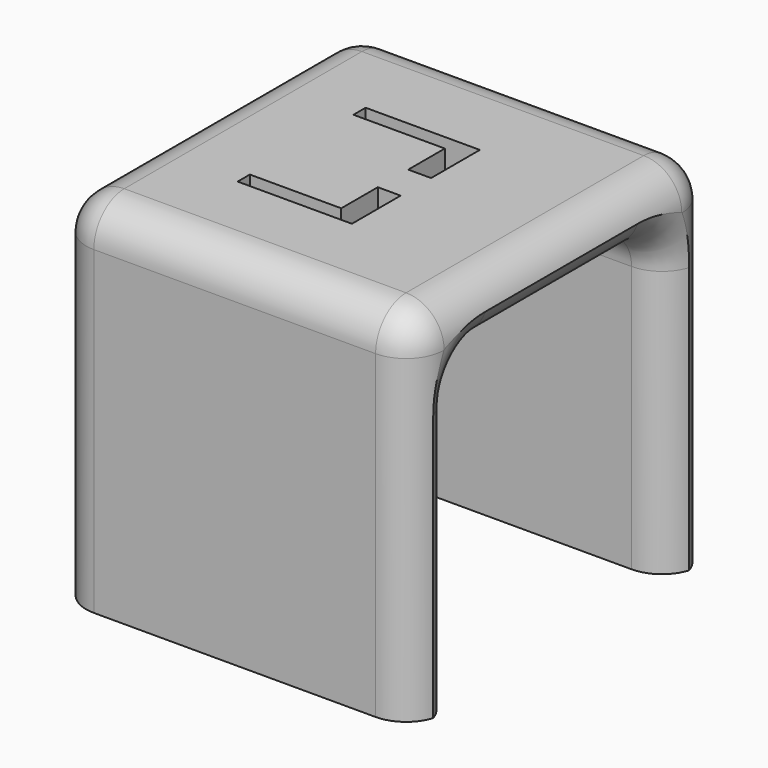
from build123d import *

# Parameters (mm, degrees)
F0_W         = 47
F0_H         = 47
F1_DEPTH     = 49
F3_DEPTH     = 40
F4_T1_DEPTH  = 37
F4_T3_DEPTH  = 54.5
F4_T5_DEPTH  = 39
F4_T7_DEPTH  = 25
F4_T9_DEPTH  = 47.5
F4_S13_W     = 5
F4_S13_H     = 5
F4_T14_DEPTH = 5
F4_S19_W     = 5
F4_S19_H     = 5
F4_T20_DEPTH = 5
F4_S25_W     = 5
F4_S25_H     = 5
F4_T26_DEPTH = 5
F4_S31_W     = 5
F4_S31_H     = 5
F4_T32_DEPTH = 5
F4_T36_ANGLE = 90
F4_T38_ANGLE = 90
F6_R         = 2.75
F7_DEPTH     = 21
F8_W         = 15
F8_H         = 21
F9_DEPTH     = 4
F10_W        = 3
F10_H        = 6
F10_W_2      = 12
F10_H_2      = 2
F11_DEPTH    = 3.0010001


# Not quite as in the source:
# - a fillet or chamfer that OpenCascade refuses, or shapes differently, is made with other operations: its cross-section is extruded or revolved along the edge and cut away or added


with BuildPart() as f1:
    # F0 (on Front) → F1 (new body)
    with BuildSketch(Plane.XZ):
        with Locations((-31.9517639409, 6.0313746929)):
            Rectangle(F0_W, F0_H)
    extrude(amount=F1_DEPTH)

    # F2 (on face) → F3 (cut)
    with BuildSketch(Plane.YZ.offset(-8.4517639409)):
        with BuildLine():
            Line((-12, 22.5313746929), (-37, 22.5313746929))
            ThreePointArc((-37, 22.5313746929), (-40.5355339059, 21.0669085988), (-42, 17.5313746929))
            Line((-42, 17.5313746929), (-42, -17.4686253071))
            Line((-42, -17.4686253071), (-7, -17.4686253071))
            Line((-7, -17.4686253071), (-7, 17.5313746929))
            ThreePointArc((-7, 17.5313746929), (-8.4644660941, 21.0669085988), (-12, 22.5313746929))
        make_face()
    extrude(amount=-F3_DEPTH, mode=Mode.SUBTRACT)

    # F4: fillet of radius 5 on 9 edges, made by hand

    # F4_s2 → F4_t1 (cut)
    with BuildSketch(Plane.YZ.offset(-50.4517639409)):
        with BuildLine():
            ThreePointArc((-44, 29.5313746929), (-47.5355339059, 28.0669085988), (-49, 24.5313746929))
            Line((-49, 24.5313746929), (-49, 29.5313746929))
            Line((-49, 29.5313746929), (-44, 29.5313746929))
        make_face()
        with BuildLine():
            ThreePointArc((0, 24.5313746929), (-1.4644660941, 28.0669085988), (-5, 29.5313746929))
            Line((-5, 29.5313746929), (0, 29.5313746929))
            Line((0, 29.5313746929), (0, 24.5313746929))
        make_face()
    extrude(amount=F4_T1_DEPTH, mode=Mode.SUBTRACT)

    # F4_s4 → F4_t3 (cut)
    with BuildSketch(Plane.XY.offset(-29.9686253071)):
        with BuildLine():
            ThreePointArc((-8.4517639409, -44), (-9.9162300349, -47.5355339059), (-13.4517639409, -49))
            Line((-13.4517639409, -49), (-8.4517639409, -49))
            Line((-8.4517639409, -49), (-8.4517639409, -44))
        make_face()
        with BuildLine():
            ThreePointArc((-8.4517639409, -5), (-9.9162300349, -1.4644660941), (-13.4517639409, 0))
            Line((-13.4517639409, 0), (-8.4517639409, 0))
            Line((-8.4517639409, 0), (-8.4517639409, -5))
        make_face()
        with BuildLine():
            ThreePointArc((-50.4517639409, 0), (-53.9872978468, -1.4644660941), (-55.4517639409, -5))
            Line((-55.4517639409, -5), (-55.4517639409, 0))
            Line((-55.4517639409, 0), (-50.4517639409, 0))
        make_face()
        with BuildLine():
            ThreePointArc((-50.4517639409, -49), (-53.9872978468, -47.5355339059), (-55.4517639409, -44))
            Line((-55.4517639409, -44), (-55.4517639409, -49))
            Line((-55.4517639409, -49), (-50.4517639409, -49))
        make_face()
    extrude(amount=F4_T3_DEPTH, mode=Mode.SUBTRACT)

    # F4_s6 → F4_t5 (cut)
    with BuildSketch(Plane.XZ.offset(5)):
        with BuildLine():
            ThreePointArc((-8.4517639409, 24.5313746929), (-9.9162300349, 28.0669085988), (-13.4517639409, 29.5313746929))
            Line((-13.4517639409, 29.5313746929), (-8.4517639409, 29.5313746929))
            Line((-8.4517639409, 29.5313746929), (-8.4517639409, 24.5313746929))
        make_face()
        with BuildLine():
            ThreePointArc((-50.4517639409, 29.5313746929), (-53.9872978468, 28.0669085988), (-55.4517639409, 24.5313746929))
            Line((-55.4517639409, 24.5313746929), (-55.4517639409, 29.5313746929))
            Line((-55.4517639409, 29.5313746929), (-50.4517639409, 29.5313746929))
        make_face()
    extrude(amount=F4_T5_DEPTH, mode=Mode.SUBTRACT)

    # F4_s8 → F4_t7 (cut)
    with BuildSketch(Plane.XZ.offset(12)):
        with BuildLine():
            ThreePointArc((-8.4517639409, 27.5313746929), (-9.9162300349, 23.995840787), (-13.4517639409, 22.5313746929))
            Line((-13.4517639409, 22.5313746929), (-8.4517639409, 22.5313746929))
            Line((-8.4517639409, 22.5313746929), (-8.4517639409, 27.5313746929))
        make_face()
    extrude(amount=F4_T7_DEPTH, mode=Mode.SUBTRACT)

    # F4_s10 → F4_t9 (cut)
    with BuildSketch(Plane.XY.offset(-29.9686253071)):
        with BuildLine():
            ThreePointArc((-8.4517639409, -47), (-9.9162300349, -43.4644660941), (-13.4517639409, -42))
            Line((-13.4517639409, -42), (-8.4517639409, -42))
            Line((-8.4517639409, -42), (-8.4517639409, -47))
        make_face()
        with BuildLine():
            ThreePointArc((-8.4517639409, -2), (-9.9162300349, -5.5355339059), (-13.4517639409, -7))
            Line((-13.4517639409, -7), (-8.4517639409, -7))
            Line((-8.4517639409, -7), (-8.4517639409, -2))
        make_face()
    extrude(amount=F4_T9_DEPTH, mode=Mode.SUBTRACT)


with BuildPart() as f4_tool12:
    # F4_s13 → F4_t14 (new body)
    with BuildSketch(Plane.YZ.offset(-13.4517639409)):
        with Locations((-46.5, 27.0313746929)):
            Rectangle(F4_S13_W, F4_S13_H)
    extrude(amount=F4_T14_DEPTH)

    # F4_s15 → F4_t16 (revolve, cut)
    with BuildSketch(Plane(origin=(-13.4517639409, -44, 24.5313746929), x_dir=(0, 0.7071067812, -0.7071067812), z_dir=(0, -0.7071067812, -0.7071067812))):
        with BuildLine():
            ThreePointArc((0, -5), (5, 0), (0, 5))
            Line((0, 5), (0, -5))
        make_face()
    revolve(axis=Axis((-13.4517639409, -44, 24.5313746929), (1, 0, 0)), mode=Mode.SUBTRACT)


with BuildPart() as f1_1:
    add(f1.part)

    # F4_t11: cut F4_tool12
    add(f4_tool12.part, mode=Mode.SUBTRACT)


with BuildPart() as f4_tool18:
    # F4_s19 → F4_t20 (new body)
    with BuildSketch(Plane.YZ.offset(-50.4517639409)):
        with Locations((-46.5, 27.0313746929)):
            Rectangle(F4_S19_W, F4_S19_H)
    extrude(amount=-F4_T20_DEPTH)

    # F4_s21 → F4_t22 (revolve, cut)
    with BuildSketch(Plane(origin=(-50.4517639409, -44, 24.5313746929), x_dir=(0, 0.7071067812, -0.7071067812), z_dir=(0, 0.7071067812, 0.7071067812))):
        with BuildLine():
            ThreePointArc((0, -5), (5, 0), (0, 5))
            Line((0, 5), (0, -5))
        make_face()
    revolve(axis=Axis((-50.4517639409, -44, 24.5313746929), (-1, 0, 0)), mode=Mode.SUBTRACT)


with BuildPart() as f1_2:
    add(f1_1.part)

    # F4_t17: cut F4_tool18
    add(f4_tool18.part, mode=Mode.SUBTRACT)


with BuildPart() as f4_tool24:
    # F4_s25 → F4_t26 (new body)
    with BuildSketch(Plane.YZ.offset(-13.4517639409)):
        with Locations((-2.5, 27.0313746929)):
            Rectangle(F4_S25_W, F4_S25_H)
    extrude(amount=F4_T26_DEPTH)

    # F4_s27 → F4_t28 (revolve, cut)
    with BuildSketch(Plane(origin=(-13.4517639409, -5, 24.5313746929), x_dir=(0, -0.7071067812, -0.7071067812), z_dir=(0, -0.7071067812, 0.7071067812))):
        with BuildLine():
            ThreePointArc((0, -5), (5, 0), (0, 5))
            Line((0, 5), (0, -5))
        make_face()
    revolve(axis=Axis((-13.4517639409, -5, 24.5313746929), (1, 0, 0)), mode=Mode.SUBTRACT)


with BuildPart() as f1_3:
    add(f1_2.part)

    # F4_t23: cut F4_tool24
    add(f4_tool24.part, mode=Mode.SUBTRACT)


with BuildPart() as f4_tool30:
    # F4_s31 → F4_t32 (new body)
    with BuildSketch(Plane.XZ.offset(5)):
        with Locations((-52.9517639409, 27.0313746929)):
            Rectangle(F4_S31_W, F4_S31_H)
    extrude(amount=-F4_T32_DEPTH)

    # F4_s33 → F4_t34 (revolve, cut)
    with BuildSketch(Plane(origin=(-50.4517639409, -5, 24.5313746929), x_dir=(0.7071067812, 0, -0.7071067812), z_dir=(0.7071067812, 0, 0.7071067812))):
        with BuildLine():
            ThreePointArc((0, -5), (5, 0), (0, 5))
            Line((0, 5), (0, -5))
        make_face()
    revolve(axis=Axis((-50.4517639409, -5, 24.5313746929), (0, 1, 0)), mode=Mode.SUBTRACT)


with BuildPart() as f1_4:
    add(f1_3.part)

    # F4_t29: cut F4_tool30
    add(f4_tool30.part, mode=Mode.SUBTRACT)

    # F4_s35 → F4_t36 (revolve, cut)
    with BuildSketch(Plane.XY.offset(17.5313746929)):
        with BuildLine():
            ThreePointArc((-8.4517639409, -2), (-9.9162300349, -5.5355339059), (-13.4517639409, -7))
            Line((-13.4517639409, -7), (-8.4517639409, -7))
            Line((-8.4517639409, -7), (-8.4517639409, -2))
        make_face()
    revolve(axis=Axis((-8.4517639409, -12, 17.5313746929), (1, 0, 0)), revolution_arc=F4_T36_ANGLE, mode=Mode.SUBTRACT)

    # F4_s37 → F4_t38 (revolve, cut)
    with BuildSketch(Plane.XZ.offset(37)):
        with BuildLine():
            ThreePointArc((-8.4517639409, 27.5313746929), (-9.9162300349, 23.995840787), (-13.4517639409, 22.5313746929))
            Line((-13.4517639409, 22.5313746929), (-8.4517639409, 22.5313746929))
            Line((-8.4517639409, 22.5313746929), (-8.4517639409, 27.5313746929))
        make_face()
    revolve(axis=Axis((-8.4517639409, -37, 17.5313746929), (1, 0, 0)), revolution_arc=F4_T38_ANGLE, mode=Mode.SUBTRACT)

    # F6 (on offset) → F7 (cut)
    with BuildSketch(Plane.XZ.offset(14.5)):
        with Locations((-45.4517639409, 24.5701503009)):
            Circle(F6_R)
    extrude(amount=F7_DEPTH, mode=Mode.SUBTRACT)

    # F8 (on face) → F9 (cut)
    with BuildSketch(Plane(origin=(0, 0, 22.5313746929), x_dir=(1, 0, 0), z_dir=(0, 0, -1))):
        with Locations((-34.8641358682, 25)):
            Rectangle(F8_W, F8_H)
    extrude(amount=-F9_DEPTH, mode=Mode.SUBTRACT)

    # F10 (on face) → F11 (cut, through all)
    with BuildSketch(Plane(origin=(0, 0, 26.5313746929), x_dir=(1, 0, 0), z_dir=(0, 0, -1))):
        with Locations((-28.8641358682, 30.5)):
            Rectangle(F10_W, F10_H)
        Polygon((-30.3641358682, 22.5), (-30.3641358682, 16.5), (-30.3641358682, 14.5), (-27.3641358682, 14.5), (-27.3641358682, 22.5), align=None)
        with Locations((-36.3641358682, 34.5)):
            Rectangle(F10_W_2, F10_H_2)
        with Locations((-28.8641358682, 34.5)):
            Rectangle(F10_W, F10_H_2)
        with Locations((-36.3641358682, 15.5)):
            Rectangle(F10_W_2, F10_H_2)
    extrude(amount=-F11_DEPTH, mode=Mode.SUBTRACT)


solid = f1_4.part
